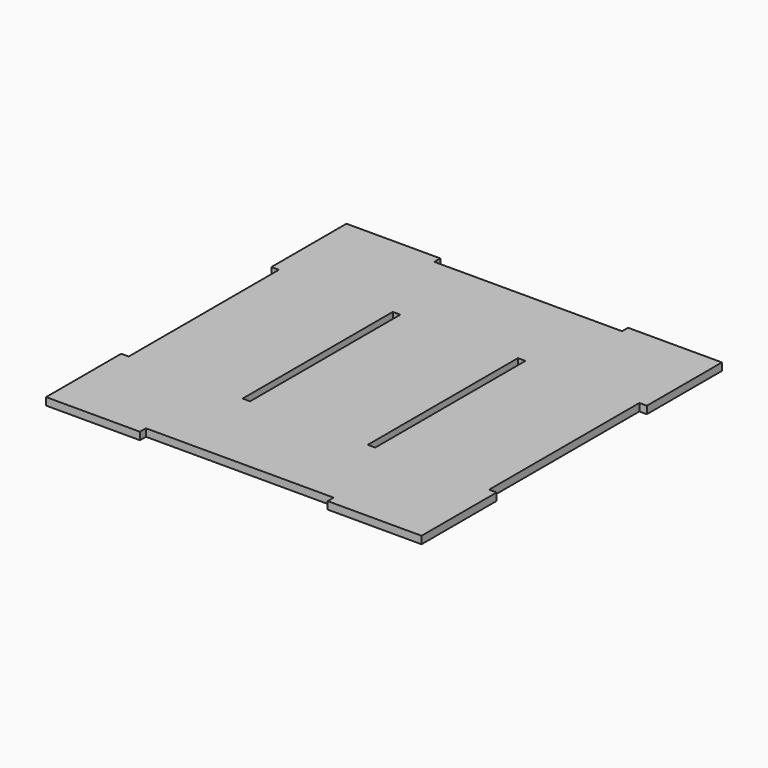
from build123d import *

# Parameters (mm, degrees)
F0_W            = 300
F0_H            = 300
F1_DEPTH        = 6
F2_W            = 150
F2_H            = 6
F3_DEPTH        = 6
F3_COPIES_COUNT = 4
F5_W            = 6
F5_H            = 150
F6_DEPTH        = 6


# Not quite as in the source:
# - a pattern or mirror of a feature is missing from the dataset's text; its kind, count and spacing are read off the source's solid


with BuildPart() as f1:
    # F0 (on Top) → F1 (new body)
    with BuildSketch(Plane.XY):
        Rectangle(F0_W, F0_H)
    extrude(amount=F1_DEPTH)

    # F2 (on face) → F3 (cut, through all)
    with BuildSketch(Plane.XY.offset(6)):
        with Locations((0, -147)):
            Rectangle(F2_W, F2_H)
    f3 = extrude(amount=-F3_DEPTH, mode=Mode.SUBTRACT)

    # F3_copies: F3 ×4 about axis
    f3_copies_axis = Axis((0, 0, 0), (0, 0, 1))
    for i in range(1, F3_COPIES_COUNT):
        add(f3.rotate(f3_copies_axis, i * 360 / F3_COPIES_COUNT), mode=Mode.SUBTRACT)

    # F5 (on face) → F6 (cut, through all)
    with BuildSketch(Plane.XY.offset(6)):
        with Locations((-50, 0)):
            Rectangle(F5_W, F5_H)
        with Locations((50, 0)):
            Rectangle(F5_W, F5_H)
    extrude(amount=-F6_DEPTH, mode=Mode.SUBTRACT)


solid = f1.part
